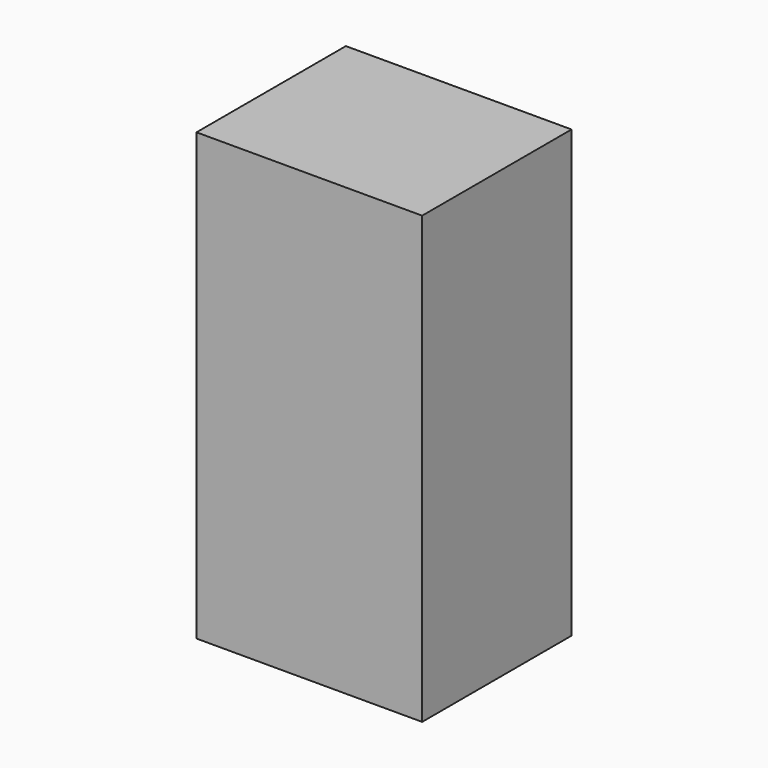
from build123d import *

# Parameters (mm, degrees)
F0_W     = 30.6968484074
F0_H     = 60.6262870133
F1_DEPTH = 25.4


# Not quite as in the source:
# - a feature names something its author has since deleted; it is built from what else it names


with BuildPart() as f1:
    # F0 (on Front) → F1 (new body)
    with BuildSketch(Plane.XZ):
        Rectangle(F0_W, F0_H)
    extrude(amount=F1_DEPTH)


solid = f1.part
